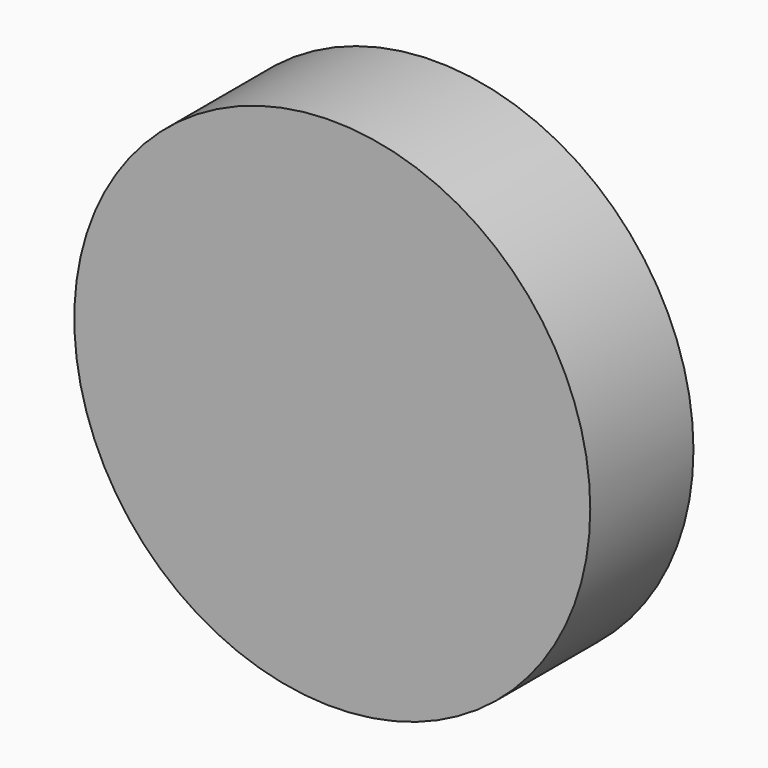
from build123d import *

# Parameters (mm, degrees)
F2_W         = 5
F2_H         = 5
F3_DEPTH     = 50.001
F4_R         = 2.499
F5_TEXT_SIZE = 34.3624161074
F6_DEPTH     = 12


# Not quite as in the source:
# - a fillet or chamfer is up to 0.001 mm smaller than in the source, because OpenCascade refuses the exact size
# - Text() gives the source's letters only with a copy of the font that has no kerning and outlines rounded to 1/6400 em; it was checked with that copy


with BuildPart() as f1:
    # F0 (on Top) → F1 (revolve)
    with BuildSketch(Plane.XY):
        Polygon((0, 5.9885961544), (0, 0), (50, 0), (50, 25), (45, 25), (45, 5.9885961544), align=None)
    revolve(axis=Axis((0, 2.9942980772, 0), (0, -1, 0)))

    # F2 (on Top) → F3 (cut, through all)
    with BuildSketch(Plane.XY):
        with Locations((0.0322200358, 22.5)):
            Rectangle(F2_W, F2_H)
    extrude(amount=-F3_DEPTH, mode=Mode.SUBTRACT)

    # F4 (radius 2.5 in the source; OpenCascade refuses exactly that, so slightly less here)
    f4_edges = [f1.edges().sort_by_distance(p)[0] for p in [
        (-2.46778, 20, -47.435673),
        (2.53222, 20, -47.432267),
    ]]
    fillet(f4_edges, radius=F4_R)

    # F5 (on face) → F6 (join)
    with BuildSketch(Plane(origin=(0, 5.9885961544, 0), x_dir=(-1, 0, 0), z_dir=(0, 1, 0))):
        with Locations((-30, -9.7409395973)):
            Text('Rot', F5_TEXT_SIZE, font='Open Sans', font_style=FontStyle.BOLD, text_align=(TextAlign.LEFT, TextAlign.BOTTOM))
    extrude(amount=F6_DEPTH)


solid = f1.part
